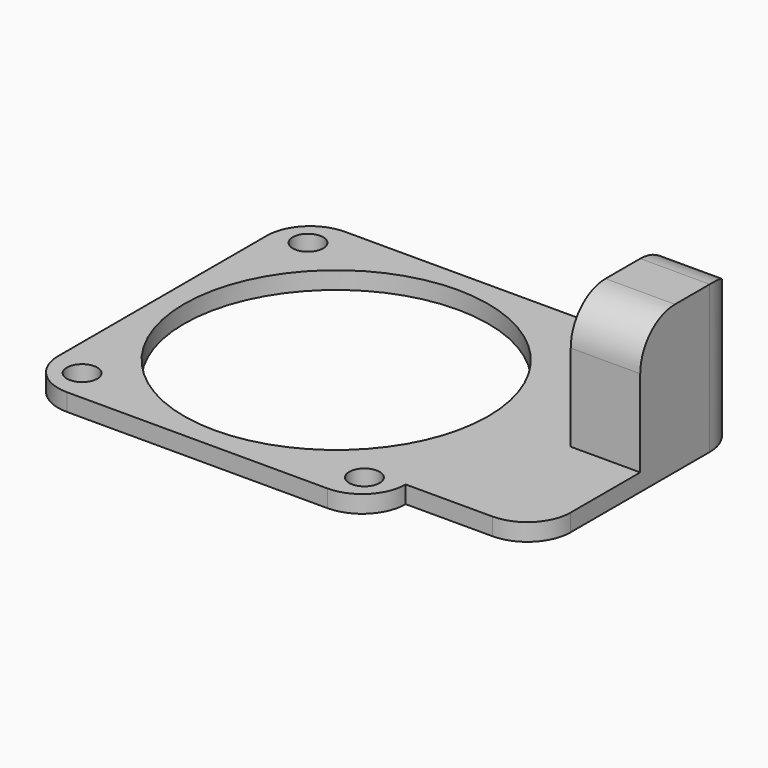
from build123d import *

# Parameters (mm, degrees)
F0_W        = 40
F0_H        = 40
F0_R        = 1.75
F0_R_2      = 17.5
F1_DEPTH    = 2
F2_R        = 5
F3_DEPTH    = 15
F4_W        = 8
F4_H        = 15
F5_DEPTH    = 15
F6_T1_DEPTH = 33
F6_T3_DEPTH = 42
F6_T5_DEPTH = 27


# Not quite as in the source:
# - a fillet or chamfer that OpenCascade refuses, or shapes differently, is made with other operations: its cross-section is extruded or revolved along the edge and cut away or added


with BuildPart() as f1:
    # F0 (on Top) → F1 (new body)
    with BuildSketch(Plane.XY):
        with Locations((9.0173190544, -26.0413483679)):
            Rectangle(F0_W, F0_H)
        with Locations((-7.2326809456, -42.2913483679)):
            Circle(F0_R, mode=Mode.SUBTRACT)
        with Locations((25.2673190544, -42.2913483679)):
            Circle(F0_R, mode=Mode.SUBTRACT)
        with Locations((9.0173190544, -26.0413483679)):
            Circle(F0_R_2, mode=Mode.SUBTRACT)
        with Locations((-7.2326809456, -9.7913483679)):
            Circle(F0_R, mode=Mode.SUBTRACT)
        with Locations((25.2673190544, -9.7913483679)):
            Circle(F0_R, mode=Mode.SUBTRACT)
    extrude(amount=F1_DEPTH)

    # F2
    f2_edges = [f1.edges().sort_by_distance(p)[0] for p in [
        (29.017319, -46.041348, 1),
        (29.017319, -6.041348, 1),
        (-10.982681, -46.041348, 1),
        (-10.982681, -6.041348, 1),
    ]]
    fillet(f2_edges, radius=F2_R)

    # F3 (add): a face of the model
    f3_faces = [f1.faces().sort_by_distance(p)[0] for p in [
        (29.0173190544, -26.0413483679, 1),
    ]]
    extrude(f3_faces, amount=F3_DEPTH)

    # F4 (on face) → F5 (join)
    with BuildSketch(Plane.XY.offset(2)):
        with Locations((40.0173190544, -18.5413483679)):
            Rectangle(F4_W, F4_H)
    extrude(amount=F5_DEPTH)

    # F6: fillet of radius 5 on 5 edges, made by hand

    # F6_s2 → F6_t1 (cut)
    with BuildSketch(Plane.YZ.offset(23.5173190544)):
        with BuildLine():
            ThreePointArc((-21.0413483679, 17), (-24.5768822739, 15.5355339059), (-26.0413483679, 12))
            Line((-26.0413483679, 12), (-26.0413483679, 17))
            Line((-26.0413483679, 17), (-21.0413483679, 17))
        make_face()
        with BuildLine():
            ThreePointArc((-16.0413483679, 17), (-12.505814462, 15.5355339059), (-11.0413483679, 12))
            Line((-11.0413483679, 12), (-11.0413483679, 17))
            Line((-11.0413483679, 17), (-16.0413483679, 17))
        make_face()
    extrude(amount=F6_T1_DEPTH, mode=Mode.SUBTRACT)

    # F6_s4 → F6_t3 (cut)
    with BuildSketch(Plane.XY.offset(-12.5)):
        with BuildLine():
            ThreePointArc((44.0173190544, -16.0413483679), (42.5528529604, -12.505814462), (39.0173190544, -11.0413483679))
            Line((39.0173190544, -11.0413483679), (44.0173190544, -11.0413483679))
            Line((44.0173190544, -11.0413483679), (44.0173190544, -16.0413483679))
        make_face()
    extrude(amount=F6_T3_DEPTH, mode=Mode.SUBTRACT)

    # F6_s6 → F6_t5 (cut)
    with BuildSketch(Plane.XY.offset(-12.5)):
        with BuildLine():
            ThreePointArc((39.0173190544, -41.0413483679), (42.5528529604, -39.5768822739), (44.0173190544, -36.0413483679))
            Line((44.0173190544, -36.0413483679), (44.0173190544, -41.0413483679))
            Line((44.0173190544, -41.0413483679), (39.0173190544, -41.0413483679))
        make_face()
    extrude(amount=F6_T5_DEPTH, mode=Mode.SUBTRACT)


solid = f1.part
